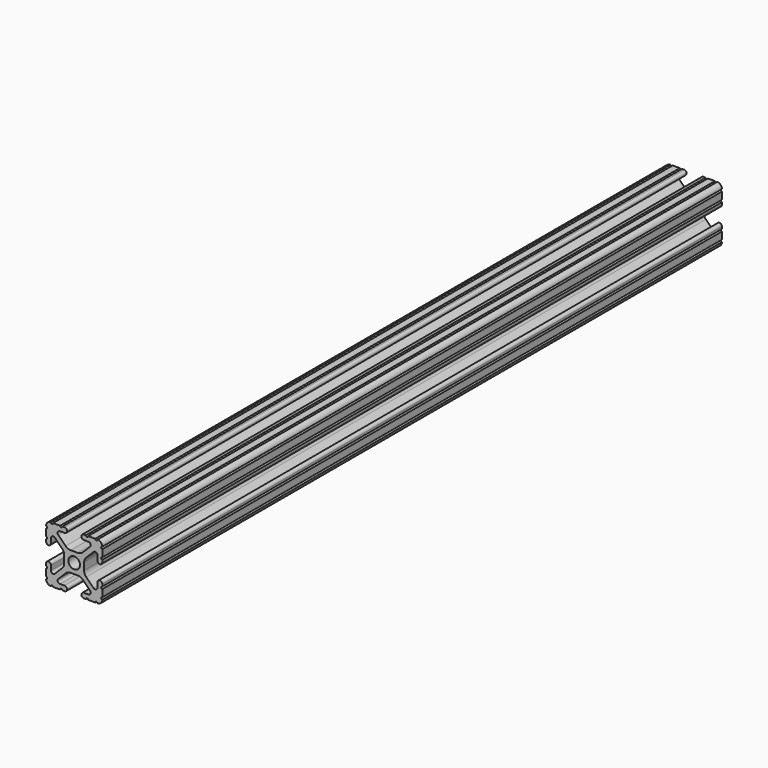
from build123d import *

# Parameters (mm, degrees)
F1_DEPTH = 375
F2_DEPTH = 25


# Not quite as in the source:
# - ends of sketch curves that miss each other by under 0.0002 mm in the source are joined


with BuildPart() as f1:
    # F0 (on Front) → F1 (new body)
    with BuildSketch(Plane.XZ):
        with BuildLine():
            ThreePointArc((-12.7, -9.5504), (-12.1920000057, -10.0583238), (-12.6998476, -10.5663999771))
            ThreePointArc((-12.6998476, -10.5663999771), (-12.0825225161, -12.0825225161), (-10.5664000074, -12.6998469825))
            ThreePointArc((-10.5664000074, -12.6998469825), (-10.0583238, -12.1920000057), (-9.5504, -12.7))
            Line((-9.5504, -12.7), (-6.3330836, -12.7))
            ThreePointArc((-6.3330836, -12.7), (-5.8250836, -12.192), (-5.3170836, -12.7))
            Line((-5.3170836, -12.7), (-4.3434, -12.7))
            ThreePointArc((-4.3434, -12.7), (-3.2385, -11.5951), (-4.3434, -10.4902))
            Line((-4.3434, -10.4902), (-6.4747902, -10.4902))
            ThreePointArc((-6.4747902, -10.4902), (-7.413451805, -9.8630063673), (-7.1932106897, -8.7557795103))
            Line((-7.1932106897, -8.7557795103), (-3.8631622, -5.4257448))
            ThreePointArc((-3.8631622, -5.4257448), (-2.8331268978, -4.7374824843), (-1.618107, -4.4958))
            Line((-1.618107, -4.4958), (1.618107, -4.4958))
            ThreePointArc((1.618107, -4.4958), (2.8331268978, -4.7374824843), (3.8631710303, -5.4257359697))
            Line((3.8631710303, -5.4257359697), (7.1932038, -8.7557864))
            ThreePointArc((7.1932038, -8.7557864), (7.413451805, -9.8630063673), (6.4747902, -10.4902))
            Line((6.4747902, -10.4902), (4.3434, -10.4902))
            ThreePointArc((4.3434, -10.4902), (3.2385, -11.5951), (4.3434, -12.7))
            Line((4.3434, -12.7), (5.3170836, -12.7))
            ThreePointArc((5.3170836, -12.7), (5.8250836, -12.192), (6.3330836, -12.7))
            Line((6.3330836, -12.7), (9.5504, -12.7))
            ThreePointArc((9.5504, -12.7), (10.0583238, -12.1920000057), (10.5663999771, -12.6998476))
            ThreePointArc((10.5663999771, -12.6998476), (12.0825225161, -12.0825225161), (12.6998469825, -10.5664000074))
            ThreePointArc((12.6998469825, -10.5664000074), (12.1920000057, -10.0583238), (12.7, -9.5504))
            Line((12.7, -9.5504), (12.7, -6.3330836))
            ThreePointArc((12.7, -6.3330836), (12.192, -5.8250836), (12.7, -5.3170836))
            Line((12.7, -5.3170836), (12.7, -4.3434))
            ThreePointArc((12.7, -4.3434), (11.5951, -3.2385), (10.4902, -4.3434))
            Line((10.4902, -4.3434), (10.4902, -6.4747902))
            ThreePointArc((10.4902, -6.4747902), (9.8630063673, -7.413451805), (8.7557795103, -7.1932106897))
            Line((8.7557795103, -7.1932106897), (5.4257448, -3.8631622))
            ThreePointArc((5.4257448, -3.8631622), (4.7374824843, -2.8331268978), (4.4958, -1.618107))
            Line((4.4958, -1.618107), (4.4958, 1.618107))
            ThreePointArc((4.4958, 1.618107), (4.7374824843, 2.8331268978), (5.4257359697, 3.8631710303))
            Line((5.4257359697, 3.8631710303), (8.7557864, 7.1932038))
            ThreePointArc((8.7557864, 7.1932038), (9.8630063673, 7.413451805), (10.4902, 6.4747902))
            Line((10.4902, 6.4747902), (10.4902, 4.3434))
            ThreePointArc((10.4902, 4.3434), (11.5951, 3.2385), (12.7, 4.3434))
            Line((12.7, 4.3434), (12.7, 5.3170836))
            ThreePointArc((12.7, 5.3170836), (12.192, 5.8250836), (12.7, 6.3330836))
            Line((12.7, 6.3330836), (12.7, 9.5504))
            ThreePointArc((12.7, 9.5504), (12.1920000057, 10.0583238), (12.6998476, 10.5663999771))
            ThreePointArc((12.6998476, 10.5663999771), (12.0825225161, 12.0825225161), (10.5664000074, 12.6998469825))
            ThreePointArc((10.5664000074, 12.6998469825), (10.0583238, 12.1920000057), (9.5504, 12.7))
            Line((9.5504, 12.7), (6.3330836, 12.7))
            ThreePointArc((6.3330836, 12.7), (5.8250836, 12.192), (5.3170836, 12.7))
            Line((5.3170836, 12.7), (4.3434, 12.7))
            ThreePointArc((4.3434, 12.7), (3.2385, 11.5951), (4.3434, 10.4902))
            Line((4.3434, 10.4902), (6.4747902, 10.4902))
            ThreePointArc((6.4747902, 10.4902), (7.413451805, 9.8630063673), (7.1932106897, 8.7557795103))
            Line((7.1932106897, 8.7557795103), (3.8631622, 5.4257448))
            ThreePointArc((3.8631622, 5.4257448), (2.8331268978, 4.7374824843), (1.618107, 4.4958))
            Line((1.618107, 4.4958), (-1.618107, 4.4958))
            ThreePointArc((-1.618107, 4.4958), (-2.8331268978, 4.7374824843), (-3.8631710303, 5.4257359697))
            Line((-3.8631710303, 5.4257359697), (-7.1932038, 8.7557864))
            ThreePointArc((-7.1932038, 8.7557864), (-7.413451805, 9.8630063673), (-6.4747902, 10.4902))
            Line((-6.4747902, 10.4902), (-4.3434, 10.4902))
            ThreePointArc((-4.3434, 10.4902), (-3.2385, 11.5951), (-4.3434, 12.7))
            Line((-4.3434, 12.7), (-5.3170836, 12.7))
            ThreePointArc((-5.3170836, 12.7), (-5.8250836, 12.192), (-6.3330836, 12.7))
            Line((-6.3330836, 12.7), (-9.5504, 12.7))
            ThreePointArc((-9.5504, 12.7), (-10.0583238, 12.1920000057), (-10.5663999771, 12.6998476))
            ThreePointArc((-10.5663999771, 12.6998476), (-12.0825225161, 12.0825225161), (-12.6998469825, 10.5664000074))
            ThreePointArc((-12.6998469825, 10.5664000074), (-12.1920000057, 10.0583238), (-12.7, 9.5504))
            Line((-12.7, 9.5504), (-12.7, 6.3330836))
            ThreePointArc((-12.7, 6.3330836), (-12.192, 5.8250836), (-12.7, 5.3170836))
            Line((-12.7, 5.3170836), (-12.7, 4.3434))
            ThreePointArc((-12.7, 4.3434), (-11.5951, 3.2385), (-10.4902, 4.3434))
            Line((-10.4902, 4.3434), (-10.4902, 6.4747902))
            ThreePointArc((-10.4902, 6.4747902), (-9.8630063673, 7.413451805), (-8.7557795103, 7.1932106897))
            Line((-8.7557795103, 7.1932106897), (-5.4257448, 3.8631622))
            ThreePointArc((-5.4257448, 3.8631622), (-4.7374824843, 2.8331268978), (-4.4958, 1.618107))
            Line((-4.4958, 1.618107), (-4.4958, -1.618107))
            ThreePointArc((-4.4958, -1.618107), (-4.7374824843, -2.8331268978), (-5.4257359697, -3.8631710303))
            Line((-5.4257359697, -3.8631710303), (-8.7557864, -7.1932038))
            ThreePointArc((-8.7557864, -7.1932038), (-9.8630063673, -7.413451805), (-10.4902, -6.4747902))
            Line((-10.4902, -6.4747902), (-10.4902, -4.3434))
            ThreePointArc((-10.4902, -4.3434), (-11.5951, -3.2385), (-12.7, -4.3434))
            Line((-12.7, -4.3434), (-12.7, -5.3170836))
            ThreePointArc((-12.7, -5.3170836), (-12.192, -5.8250836), (-12.7, -6.3330836))
            Line((-12.7, -6.3330836), (-12.7, -9.5504))
        make_face()
        with BuildLine():
            ThreePointArc((-2.6035, 0), (0, 2.6035), (2.6035, 0))
            ThreePointArc((2.6035, 0), (0, -2.6035), (-2.6035, 0))
        make_face(mode=Mode.SUBTRACT)
    extrude(amount=F1_DEPTH)

    # F2 (cut): a face of the model
    f2_faces = [f1.faces().sort_by_distance(p)[0] for p in [
        (-10.849410262, -375, 5.4090951),
    ]]
    extrude(f2_faces, amount=-F2_DEPTH, mode=Mode.SUBTRACT)


solid = f1.part
